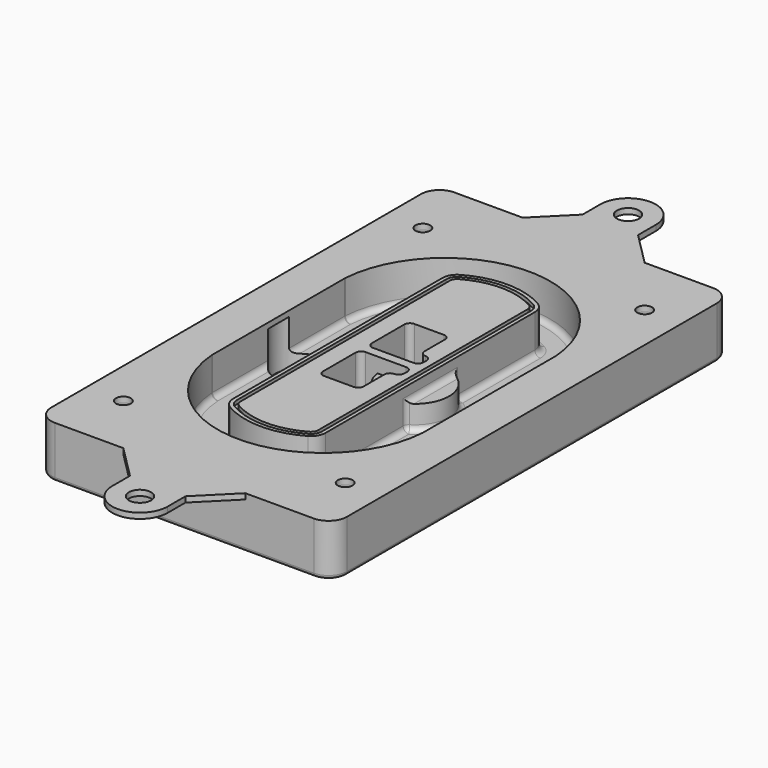
from build123d import *

# Parameters (mm, degrees)
F0_R      = 4
F1_DEPTH  = 25
F2_DEPTH  = 3
F3_DEPTH  = 18
F5_DEPTH  = 21
F6_DEPTH  = 2
F8_DEPTH  = 20
F9_DEPTH  = 16
F10_DEPTH = 25
F7_R      = 6
F7_R_2    = 4
F11_DEPTH = 6
F13_DEPTH = 9
F14_R     = 3
F15_R     = 2
F16_R     = 4
F16_R_2   = 6
F17_DEPTH = 3


with BuildPart() as f1:
    # F0 (on Top) → F1 (new body)
    with BuildSketch(Plane.XY):
        with BuildLine():
            ThreePointArc((-80, -125), (-77.0710678119, -132.0710678119), (-70, -135))
            Line((-70, -135), (70, -135))
            ThreePointArc((70, -135), (77.0710678119, -132.0710678119), (80, -125))
            Line((80, -125), (80, 125))
            ThreePointArc((80, 125), (77.0710678119, 132.0710678119), (70, 135))
            Line((70, 135), (-70, 135))
            ThreePointArc((-70, 135), (-77.0710678119, 132.0710678119), (-80, 125))
            Line((-80, 125), (-80, -125))
        make_face()
        with Locations((-60, -101.25)):
            Circle(F0_R, mode=Mode.SUBTRACT)
        with Locations((60, -101.25)):
            Circle(F0_R, mode=Mode.SUBTRACT)
        with Locations((-60, 101.25)):
            Circle(F0_R, mode=Mode.SUBTRACT)
        with BuildLine():
            ThreePointArc((-64, 44.6627429245), (-63.991269098, 45.1571001106), (-63.9650872818, 45.650840699))
            ThreePointArc((-63.9650872818, 45.650840699), (0, 105.25), (63.9650872818, 45.650840699))
            ThreePointArc((63.9650872818, 45.650840699), (63.991269098, 45.1571001106), (64, 44.6627429245))
            Line((64, 44.6627429245), (64, -44.6627429245))
            ThreePointArc((64, -44.6627429245), (63.991269098, -45.1571001106), (63.9650872818, -45.650840699))
            ThreePointArc((63.9650872818, -45.650840699), (0, -105.25), (-63.9650872818, -45.650840699))
            ThreePointArc((-63.9650872818, -45.650840699), (-63.991269098, -45.1571001106), (-64, -44.6627429245))
            Line((-64, -44.6627429245), (-64, 44.6627429245))
        make_face(mode=Mode.SUBTRACT)
        with Locations((60, 101.25)):
            Circle(F0_R, mode=Mode.SUBTRACT)
        with BuildLine():
            ThreePointArc((63.9650872818, 45.650840699), (0, 105.25), (-63.9650872818, 45.650840699))
            ThreePointArc((-63.9650872818, 45.650840699), (-63.991269098, 45.1571001106), (-64, 44.6627429245))
            Line((-64, 44.6627429245), (-64, -44.6627429245))
            ThreePointArc((-64, -44.6627429245), (-63.991269098, -45.1571001106), (-63.9650872818, -45.650840699))
            ThreePointArc((-63.9650872818, -45.650840699), (0, -105.25), (63.9650872818, -45.650840699))
            ThreePointArc((63.9650872818, -45.650840699), (63.991269098, -45.1571001106), (64, -44.6627429245))
            Line((64, -44.6627429245), (64, 44.6627429245))
            ThreePointArc((64, 44.6627429245), (63.991269098, 45.1571001106), (63.9650872818, 45.650840699))
        make_face()
        with BuildLine():
            Line((-60, -44.6627429245), (-60, 44.6627429245))
            ThreePointArc((-60, 44.6627429245), (-59.9937636414, 45.0158552003), (-59.9750623441, 45.3685270491))
            ThreePointArc((-59.9750623441, 45.3685270491), (0, 101.25), (59.9750623441, 45.3685270491))
            ThreePointArc((59.9750623441, 45.3685270491), (59.9937636414, 45.0158552003), (60, 44.6627429245))
            Line((60, 44.6627429245), (60, -44.6627429245))
            ThreePointArc((60, -44.6627429245), (59.9937636414, -45.0158552003), (59.9750623441, -45.3685270491))
            ThreePointArc((59.9750623441, -45.3685270491), (0, -101.25), (-59.9750623441, -45.3685270491))
            ThreePointArc((-59.9750623441, -45.3685270491), (-59.9937636414, -45.0158552003), (-60, -44.6627429245))
        make_face(mode=Mode.SUBTRACT)
        with BuildLine():
            ThreePointArc((-59.9750623441, 45.3685270491), (-59.9937636414, 45.0158552003), (-60, 44.6627429245))
            Line((-60, 44.6627429245), (-60, -44.6627429245))
            ThreePointArc((-60, -44.6627429245), (-59.9937636414, -45.0158552003), (-59.9750623441, -45.3685270491))
            ThreePointArc((-59.9750623441, -45.3685270491), (0, -101.25), (59.9750623441, -45.3685270491))
            ThreePointArc((59.9750623441, -45.3685270491), (59.9937636414, -45.0158552003), (60, -44.6627429245))
            Line((60, -44.6627429245), (60, 44.6627429245))
            ThreePointArc((60, 44.6627429245), (59.9937636414, 45.0158552003), (59.9750623441, 45.3685270491))
            ThreePointArc((59.9750623441, 45.3685270491), (0, 101.25), (-59.9750623441, 45.3685270491))
        make_face()
        with BuildLine():
            ThreePointArc((56.9825436409, 45.1567918117), (56.995634549, 44.9099215176), (57, 44.6627429245))
            Line((57, 44.6627429245), (57, -44.6627429245))
            ThreePointArc((57, -44.6627429245), (56.995634549, -44.9099215176), (56.9825436409, -45.1567918117))
            ThreePointArc((56.9825436409, -45.1567918117), (0, -98.25), (-56.9825436409, -45.1567918117))
            ThreePointArc((-56.9825436409, -45.1567918117), (-56.995634549, -44.9099215176), (-57, -44.6627429245))
            Line((-57, -44.6627429245), (-57, 44.6627429245))
            ThreePointArc((-57, 44.6627429245), (-56.995634549, 44.9099215176), (-56.9825436409, 45.1567918117))
            ThreePointArc((-56.9825436409, 45.1567918117), (0, 98.25), (56.9825436409, 45.1567918117))
        make_face(mode=Mode.SUBTRACT)
        with BuildLine():
            Line((57, -44.6627429245), (57, 44.6627429245))
            ThreePointArc((57, 44.6627429245), (56.995634549, 44.9099215176), (56.9825436409, 45.1567918117))
            ThreePointArc((56.9825436409, 45.1567918117), (0, 98.25), (-56.9825436409, 45.1567918117))
            ThreePointArc((-56.9825436409, 45.1567918117), (-56.995634549, 44.9099215176), (-57, 44.6627429245))
            Line((-57, 44.6627429245), (-57, -44.6627429245))
            ThreePointArc((-57, -44.6627429245), (-56.995634549, -44.9099215176), (-56.9825436409, -45.1567918117))
            ThreePointArc((-56.9825436409, -45.1567918117), (0, -98.25), (56.9825436409, -45.1567918117))
            ThreePointArc((56.9825436409, -45.1567918117), (56.995634549, -44.9099215176), (57, -44.6627429245))
        make_face()
    extrude(amount=-F1_DEPTH)

    # F0 (on Top) → F2 (join)
    with BuildSketch(Plane.XY):
        with BuildLine():
            ThreePointArc((-59.9750623441, 45.3685270491), (-59.9937636414, 45.0158552003), (-60, 44.6627429245))
            Line((-60, 44.6627429245), (-60, -44.6627429245))
            ThreePointArc((-60, -44.6627429245), (-59.9937636414, -45.0158552003), (-59.9750623441, -45.3685270491))
            ThreePointArc((-59.9750623441, -45.3685270491), (0, -101.25), (59.9750623441, -45.3685270491))
            ThreePointArc((59.9750623441, -45.3685270491), (59.9937636414, -45.0158552003), (60, -44.6627429245))
            Line((60, -44.6627429245), (60, 44.6627429245))
            ThreePointArc((60, 44.6627429245), (59.9937636414, 45.0158552003), (59.9750623441, 45.3685270491))
            ThreePointArc((59.9750623441, 45.3685270491), (0, 101.25), (-59.9750623441, 45.3685270491))
        make_face()
        with BuildLine():
            ThreePointArc((56.9825436409, 45.1567918117), (56.995634549, 44.9099215176), (57, 44.6627429245))
            Line((57, 44.6627429245), (57, -44.6627429245))
            ThreePointArc((57, -44.6627429245), (56.995634549, -44.9099215176), (56.9825436409, -45.1567918117))
            ThreePointArc((56.9825436409, -45.1567918117), (0, -98.25), (-56.9825436409, -45.1567918117))
            ThreePointArc((-56.9825436409, -45.1567918117), (-56.995634549, -44.9099215176), (-57, -44.6627429245))
            Line((-57, -44.6627429245), (-57, 44.6627429245))
            ThreePointArc((-57, 44.6627429245), (-56.995634549, 44.9099215176), (-56.9825436409, 45.1567918117))
            ThreePointArc((-56.9825436409, 45.1567918117), (0, 98.25), (56.9825436409, 45.1567918117))
        make_face(mode=Mode.SUBTRACT)
    extrude(amount=F2_DEPTH)

    # F0 (on Top) → F3 (cut)
    with BuildSketch(Plane.XY):
        with BuildLine():
            Line((57, -44.6627429245), (57, 44.6627429245))
            ThreePointArc((57, 44.6627429245), (56.995634549, 44.9099215176), (56.9825436409, 45.1567918117))
            ThreePointArc((56.9825436409, 45.1567918117), (0, 98.25), (-56.9825436409, 45.1567918117))
            ThreePointArc((-56.9825436409, 45.1567918117), (-56.995634549, 44.9099215176), (-57, 44.6627429245))
            Line((-57, 44.6627429245), (-57, -44.6627429245))
            ThreePointArc((-57, -44.6627429245), (-56.995634549, -44.9099215176), (-56.9825436409, -45.1567918117))
            ThreePointArc((-56.9825436409, -45.1567918117), (0, -98.25), (56.9825436409, -45.1567918117))
            ThreePointArc((56.9825436409, -45.1567918117), (56.995634549, -44.9099215176), (57, -44.6627429245))
        make_face()
    extrude(amount=-F3_DEPTH, mode=Mode.SUBTRACT)

    # F4 (on face) → F5 (join, through all)
    with BuildSketch(Plane.XY.offset(3)):
        with BuildLine():
            ThreePointArc((-25, -70.7141132851), (-23.9239722661, -74.7214325959), (-20.9853479853, -77.6507552274))
            ThreePointArc((-20.9853479853, -77.6507552274), (0, -83.25), (20.9853479853, -77.6507552274))
            ThreePointArc((20.9853479853, -77.6507552274), (23.9239722661, -74.7214325959), (25, -70.7141132851))
            Line((25, -70.7141132851), (25, 70.7141132851))
            ThreePointArc((25, 70.7141132851), (23.9239722661, 74.7214325959), (20.9853479853, 77.6507552274))
            ThreePointArc((20.9853479853, 77.6507552274), (0, 83.25), (-20.9853479853, 77.6507552274))
            ThreePointArc((-20.9853479853, 77.6507552274), (-23.9239722661, 74.7214325959), (-25, 70.7141132851))
            Line((-25, 70.7141132851), (-25, -70.7141132851))
        make_face()
        with BuildLine():
            ThreePointArc((19.989010989, 75.9165947419), (22.1929791996, 73.7196027682), (23, 70.7141132851))
            Line((23, 70.7141132851), (23, -70.7141132851))
            ThreePointArc((23, -70.7141132851), (22.1929791996, -73.7196027682), (19.989010989, -75.9165947419))
            ThreePointArc((19.989010989, -75.9165947419), (0, -81.25), (-19.989010989, -75.9165947419))
            ThreePointArc((-19.989010989, -75.9165947419), (-22.1929791996, -73.7196027682), (-23, -70.7141132851))
            Line((-23, -70.7141132851), (-23, 70.7141132851))
            ThreePointArc((-23, 70.7141132851), (-22.1929791996, 73.7196027682), (-19.989010989, 75.9165947419))
            ThreePointArc((-19.989010989, 75.9165947419), (0, 81.25), (19.989010989, 75.9165947419))
        make_face(mode=Mode.SUBTRACT)
        with BuildLine():
            Line((23, -70.7141132851), (23, 70.7141132851))
            ThreePointArc((23, 70.7141132851), (22.1929791996, 73.7196027682), (19.989010989, 75.9165947419))
            ThreePointArc((19.989010989, 75.9165947419), (0, 81.25), (-19.989010989, 75.9165947419))
            ThreePointArc((-19.989010989, 75.9165947419), (-22.1929791996, 73.7196027682), (-23, 70.7141132851))
            Line((-23, 70.7141132851), (-23, -70.7141132851))
            ThreePointArc((-23, -70.7141132851), (-22.1929791996, -73.7196027682), (-19.989010989, -75.9165947419))
            ThreePointArc((-19.989010989, -75.9165947419), (0, -81.25), (19.989010989, -75.9165947419))
            ThreePointArc((19.989010989, -75.9165947419), (22.1929791996, -73.7196027682), (23, -70.7141132851))
        make_face()
        with BuildLine():
            ThreePointArc((18.9926739927, 74.1824342563), (20.461986133, 72.7177729405), (21, 70.7141132851))
            Line((21, 70.7141132851), (21, -70.7141132851))
            ThreePointArc((21, -70.7141132851), (20.461986133, -72.7177729405), (18.9926739927, -74.1824342563))
            ThreePointArc((18.9926739927, -74.1824342563), (0, -79.25), (-18.9926739927, -74.1824342563))
            ThreePointArc((-18.9926739927, -74.1824342563), (-20.461986133, -72.7177729405), (-21, -70.7141132851))
            Line((-21, -70.7141132851), (-21, 70.7141132851))
            ThreePointArc((-21, 70.7141132851), (-20.461986133, 72.7177729405), (-18.9926739927, 74.1824342563))
            ThreePointArc((-18.9926739927, 74.1824342563), (0, 79.25), (18.9926739927, 74.1824342563))
        make_face(mode=Mode.SUBTRACT)
        with BuildLine():
            Line((21, -70.7141132851), (21, 70.7141132851))
            ThreePointArc((21, 70.7141132851), (20.461986133, 72.7177729405), (18.9926739927, 74.1824342563))
            ThreePointArc((18.9926739927, 74.1824342563), (0, 79.25), (-18.9926739927, 74.1824342563))
            ThreePointArc((-18.9926739927, 74.1824342563), (-20.461986133, 72.7177729405), (-21, 70.7141132851))
            Line((-21, 70.7141132851), (-21, -70.7141132851))
            ThreePointArc((-21, -70.7141132851), (-20.461986133, -72.7177729405), (-18.9926739927, -74.1824342563))
            ThreePointArc((-18.9926739927, -74.1824342563), (0, -79.25), (18.9926739927, -74.1824342563))
            ThreePointArc((18.9926739927, -74.1824342563), (20.461986133, -72.7177729405), (21, -70.7141132851))
        make_face()
        with BuildLine():
            Line((-8, -2.5), (14, -2.5))
            ThreePointArc((14, -2.5), (16.1213203436, -3.3786796564), (17, -5.5))
            Line((17, -5.5), (17, -7.5))
            ThreePointArc((17, -7.5), (16.1213203436, -9.6213203436), (14, -10.5))
            ThreePointArc((14, -10.5), (11.8786796564, -11.3786796564), (11, -13.5))
            Line((11, -13.5), (11, -27.5))
            ThreePointArc((11, -27.5), (10.1213203436, -29.6213203436), (8, -30.5))
            Line((8, -30.5), (-8, -30.5))
            ThreePointArc((-8, -30.5), (-10.1213203436, -29.6213203436), (-11, -27.5))
            Line((-11, -27.5), (-11, -5.5))
            ThreePointArc((-11, -5.5), (-10.1213203436, -3.3786796564), (-8, -2.5))
        make_face(mode=Mode.SUBTRACT)
        with BuildLine():
            ThreePointArc((-8, 2.5), (-10.1213203436, 3.3786796564), (-11, 5.5))
            Line((-11, 5.5), (-11, 27.5))
            ThreePointArc((-11, 27.5), (-10.1213203436, 29.6213203436), (-8, 30.5))
            Line((-8, 30.5), (8, 30.5))
            ThreePointArc((8, 30.5), (10.1213203436, 29.6213203436), (11, 27.5))
            Line((11, 27.5), (11, 13.5))
            ThreePointArc((11, 13.5), (11.8786796564, 11.3786796564), (14, 10.5))
            ThreePointArc((14, 10.5), (16.1213203436, 9.6213203436), (17, 7.5))
            Line((17, 7.5), (17, 5.5))
            ThreePointArc((17, 5.5), (16.1213203436, 3.3786796564), (14, 2.5))
            Line((14, 2.5), (-8, 2.5))
        make_face(mode=Mode.SUBTRACT)
    extrude(amount=-F5_DEPTH)

    # F4 (on face) → F6 (cut)
    with BuildSketch(Plane.XY.offset(3)):
        with BuildLine():
            Line((23, -70.7141132851), (23, 70.7141132851))
            ThreePointArc((23, 70.7141132851), (22.1929791996, 73.7196027682), (19.989010989, 75.9165947419))
            ThreePointArc((19.989010989, 75.9165947419), (0, 81.25), (-19.989010989, 75.9165947419))
            ThreePointArc((-19.989010989, 75.9165947419), (-22.1929791996, 73.7196027682), (-23, 70.7141132851))
            Line((-23, 70.7141132851), (-23, -70.7141132851))
            ThreePointArc((-23, -70.7141132851), (-22.1929791996, -73.7196027682), (-19.989010989, -75.9165947419))
            ThreePointArc((-19.989010989, -75.9165947419), (0, -81.25), (19.989010989, -75.9165947419))
            ThreePointArc((19.989010989, -75.9165947419), (22.1929791996, -73.7196027682), (23, -70.7141132851))
        make_face()
        with BuildLine():
            ThreePointArc((18.9926739927, 74.1824342563), (20.461986133, 72.7177729405), (21, 70.7141132851))
            Line((21, 70.7141132851), (21, -70.7141132851))
            ThreePointArc((21, -70.7141132851), (20.461986133, -72.7177729405), (18.9926739927, -74.1824342563))
            ThreePointArc((18.9926739927, -74.1824342563), (0, -79.25), (-18.9926739927, -74.1824342563))
            ThreePointArc((-18.9926739927, -74.1824342563), (-20.461986133, -72.7177729405), (-21, -70.7141132851))
            Line((-21, -70.7141132851), (-21, 70.7141132851))
            ThreePointArc((-21, 70.7141132851), (-20.461986133, 72.7177729405), (-18.9926739927, 74.1824342563))
            ThreePointArc((-18.9926739927, 74.1824342563), (0, 79.25), (18.9926739927, 74.1824342563))
        make_face(mode=Mode.SUBTRACT)
    extrude(amount=-F6_DEPTH, mode=Mode.SUBTRACT)

    # F7 (on face) → F8 (join)
    with BuildSketch(Plane(origin=(0, 0, -25), x_dir=(1, 0, 0), z_dir=(0, 0, -1))):
        with BuildLine():
            ThreePointArc((3.28842436, 0), (16.7567035675, 13.4682792075), (30.224982775, 0))
            Line((30.224982775, 0), (35.224982775, 0))
            ThreePointArc((35.224982775, 0), (16.7567035675, 18.4682792075), (-1.71157564, 0))
            Line((-1.71157564, 0), (3.28842436, 0))
        make_face()
        with BuildLine():
            Line((3.28842436, 0), (30.224982775, 0))
            ThreePointArc((30.224982775, 0), (16.7567035675, 13.4682792075), (3.28842436, 0))
        make_face()
        with BuildLine():
            ThreePointArc((3.28842436, 0), (16.7567035675, -13.4682792075), (30.224982775, 0))
            Line((30.224982775, 0), (3.28842436, 0))
        make_face()
        with BuildLine():
            Line((35.224982775, 0), (30.224982775, 0))
            ThreePointArc((30.224982775, 0), (16.7567035675, -13.4682792075), (3.28842436, 0))
            Line((3.28842436, 0), (-1.71157564, 0))
            ThreePointArc((-1.71157564, 0), (16.7567035675, -18.4682792075), (35.224982775, 0))
        make_face()
    extrude(amount=-F8_DEPTH)

    # F7 (on face) → F9 (cut)
    with BuildSketch(Plane(origin=(0, 0, -25), x_dir=(1, 0, 0), z_dir=(0, 0, -1))):
        with BuildLine():
            Line((3.28842436, 0), (30.224982775, 0))
            ThreePointArc((30.224982775, 0), (16.7567035675, 13.4682792075), (3.28842436, 0))
        make_face()
        with BuildLine():
            ThreePointArc((3.28842436, 0), (16.7567035675, -13.4682792075), (30.224982775, 0))
            Line((30.224982775, 0), (3.28842436, 0))
        make_face()
    extrude(amount=-F9_DEPTH, mode=Mode.SUBTRACT)

    # F7 (on face) → F10 (cut)
    with BuildSketch(Plane(origin=(0, 0, -25), x_dir=(1, 0, 0), z_dir=(0, 0, -1))):
        with BuildLine():
            Line((-59.0318229325, 0), (-32.0952645175, 0))
            ThreePointArc((-32.0952645175, 0), (-45.563543725, 13.4682792075), (-59.0318229325, 0))
        make_face()
        with BuildLine():
            ThreePointArc((-59.0318229325, 0), (-45.563543725, -13.4682792075), (-32.0952645175, 0))
            Line((-32.0952645175, 0), (-59.0318229325, 0))
        make_face()
    extrude(amount=-F10_DEPTH, mode=Mode.SUBTRACT)

    # F7 (on face) → F11 (cut)
    with BuildSketch(Plane(origin=(0, 0, -25), x_dir=(1, 0, 0), z_dir=(0, 0, -1))):
        with Locations((60, -101.25)):
            Circle(F7_R)
        with Locations((60, -101.25)):
            Circle(F7_R_2, mode=Mode.SUBTRACT)
        with Locations((-60, -101.25)):
            Circle(F7_R)
        with Locations((-60, -101.25)):
            Circle(F7_R_2, mode=Mode.SUBTRACT)
        with Locations((-60, 101.25)):
            Circle(F7_R)
        with Locations((-60, 101.25)):
            Circle(F7_R_2, mode=Mode.SUBTRACT)
        with Locations((60, 101.25)):
            Circle(F7_R)
        with Locations((60, 101.25)):
            Circle(F7_R_2, mode=Mode.SUBTRACT)
    extrude(amount=-F11_DEPTH, mode=Mode.SUBTRACT)

    # F12 (on face) → F13 (cut, through all)
    with BuildSketch(Plane(origin=(0, 0, -9), x_dir=(1, 0, 0), z_dir=(0, 0, -1))):
        with BuildLine():
            Line((11, 13.5), (11, 17.5481537753))
            ThreePointArc((11, 17.5481537753), (2.5696536419, 11.8239143813), (-1.5415842455, 2.5))
            Line((-1.5415842455, 2.5), (3.5224848595, 2.5))
            ThreePointArc((3.5224848595, 2.5), (6.1857188154, 8.3455872281), (11.2536447004, 12.2927168648))
            ThreePointArc((11.2536447004, 12.2927168648), (11.0640958889, 12.8831798879), (11, 13.5))
        make_face()
        with BuildLine():
            ThreePointArc((11.2536447004, -12.2927168648), (6.1857188154, -8.3455872281), (3.5224848595, -2.5))
            Line((3.5224848595, -2.5), (-1.5415842455, -2.5))
            ThreePointArc((-1.5415842455, -2.5), (2.5696536419, -11.8239143813), (11, -17.5481537753))
            Line((11, -17.5481537753), (11, -13.5))
            ThreePointArc((11, -13.5), (11.0640958889, -12.8831798879), (11.2536447004, -12.2927168648))
        make_face()
        with BuildLine():
            ThreePointArc((11.2536447004, 12.2927168648), (6.1857188154, 8.3455872281), (3.5224848595, 2.5))
            Line((3.5224848595, 2.5), (14, 2.5))
            ThreePointArc((14, 2.5), (16.1213203436, 3.3786796564), (17, 5.5))
            Line((17, 5.5), (17, 7.5))
            ThreePointArc((17, 7.5), (16.1213203436, 9.6213203436), (14, 10.5))
            ThreePointArc((14, 10.5), (12.3601599782, 10.9878446101), (11.2536447004, 12.2927168648))
        make_face()
        with BuildLine():
            Line((14, -2.5), (3.5224848595, -2.5))
            ThreePointArc((3.5224848595, -2.5), (6.1857188154, -8.3455872281), (11.2536447004, -12.2927168648))
            ThreePointArc((11.2536447004, -12.2927168648), (12.3601599782, -10.9878446101), (14, -10.5))
            ThreePointArc((14, -10.5), (16.1213203436, -9.6213203436), (17, -7.5))
            Line((17, -7.5), (17, -5.5))
            ThreePointArc((17, -5.5), (16.1213203436, -3.3786796564), (14, -2.5))
        make_face()
    extrude(amount=F13_DEPTH, mode=Mode.SUBTRACT)

    # F14
    f14_edges = [f1.edges().sort_by_distance(p)[0] for p in [
        (-57, -25.888126, -18),
        (-57, 25.888126, -18),
        (25, 0, -5),
        (25, 16.526506, -11.5),
        (25, -16.526506, -11.5),
        (25, -43.62031, -18),
        (35.224983, 0, -18),
    ]]
    fillet(f14_edges, radius=F14_R)

    # F15
    f15_edges = [f1.edges().sort_by_distance(p)[0] for p in [
        (0, -135, -25),
    ]]
    fillet(f15_edges, radius=F15_R)

    # F16 (on face) → F17 (join, through all)
    with BuildSketch(Plane.XY):
        with BuildLine():
            Line((33, -135), (70, -135))
            ThreePointArc((70, -135), (77.0710678119, -132.0710678119), (80, -125))
            Line((80, -125), (80, 125))
            ThreePointArc((80, 125), (77.0710678119, 132.0710678119), (70, 135))
            Line((70, 135), (33, 135))
            Line((33, 135), (-33, 135))
            Line((-33, 135), (-70, 135))
            ThreePointArc((-70, 135), (-77.0710678119, 132.0710678119), (-80, 125))
            Line((-80, 125), (-80, -125))
            ThreePointArc((-80, -125), (-77.0710678119, -132.0710678119), (-70, -135))
            Line((-70, -135), (-33, -135))
            Line((-33, -135), (33, -135))
        make_face()
        with Locations((-60, -101.25)):
            Circle(F16_R, mode=Mode.SUBTRACT)
        with Locations((60, -101.25)):
            Circle(F16_R, mode=Mode.SUBTRACT)
        with Locations((-60, 101.25)):
            Circle(F16_R, mode=Mode.SUBTRACT)
        with BuildLine():
            Line((-60, -44.6627429245), (-60, 44.6627429245))
            ThreePointArc((-60, 44.6627429245), (-59.9937636414, 45.0158552003), (-59.9750623441, 45.3685270491))
            ThreePointArc((-59.9750623441, 45.3685270491), (0, 101.25), (59.9750623441, 45.3685270491))
            ThreePointArc((59.9750623441, 45.3685270491), (59.9937636414, 45.0158552003), (60, 44.6627429245))
            Line((60, 44.6627429245), (60, -44.6627429245))
            ThreePointArc((60, -44.6627429245), (59.9937636414, -45.0158552003), (59.9750623441, -45.3685270491))
            ThreePointArc((59.9750623441, -45.3685270491), (0, -101.25), (-59.9750623441, -45.3685270491))
            ThreePointArc((-59.9750623441, -45.3685270491), (-59.9937636414, -45.0158552003), (-60, -44.6627429245))
        make_face(mode=Mode.SUBTRACT)
        with Locations((60, 101.25)):
            Circle(F16_R, mode=Mode.SUBTRACT)
        with BuildLine():
            Line((15, -153), (33, -135))
            Line((33, -135), (-33, -135))
            Line((-33, -135), (-15, -153))
            Line((-15, -153), (-15, -165))
            ThreePointArc((-15, -165), (0, -180), (15, -165))
            Line((15, -165), (15, -153))
        make_face()
        with Locations((0, -165)):
            Circle(F16_R_2, mode=Mode.SUBTRACT)
        with BuildLine():
            Line((-33, 135), (33, 135))
            Line((33, 135), (15, 153))
            Line((15, 153), (15, 165))
            ThreePointArc((15, 165), (0, 180), (-15, 165))
            Line((-15, 165), (-15, 153))
            Line((-15, 153), (-33, 135))
        make_face()
        with Locations((0, 165)):
            Circle(F16_R_2, mode=Mode.SUBTRACT)
    extrude(amount=F17_DEPTH)


solid = f1.part
